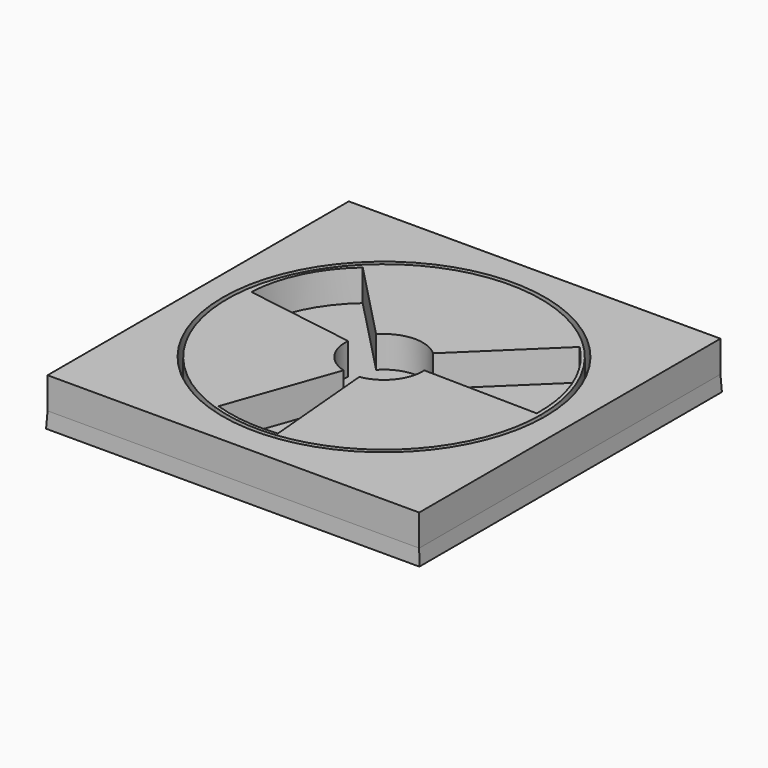
from build123d import *

# Parameters (mm, degrees)
F1_DEPTH  = 12.7
F0_R      = 72.898
F0_R_2    = 65.278
F2_DEPTH  = 12.7
F4_R      = 72.898
F5_DEPTH  = 6.35
F6_DEPTH  = 12.7
F8_W      = 150.4707932472
F8_H      = 152.4543464184
F8_R      = 72.898
F9_DEPTH  = 12.7
F9_FACE_W = 150.4707932472
F9_FACE_H = 152.4543464184
F9_FACE_R = 72.898
F12_DEPTH = 6.35
F12_TAPER = -3


# Not quite as in the source:
# - the program builds the solid bodies; features that only make, move or delete a surface that nothing else refers to are left out


with BuildPart() as f1:
    # F0 (on Top) → F1 (new body)
    with BuildSketch(Plane.XY):
        with BuildLine():
            Line((44.0266140713, 43.9798835084), (44.9402432342, 44.8622841377))
            ThreePointArc((44.9402432342, 44.8622841377), (0.0822011404, 63.499946795), (-44.8239437094, 44.9784845269))
            Line((-44.8239437094, 44.9784845269), (-43.499038361, 43.6043470536))
            Line((-43.499038361, 43.6043470536), (-11.6539793168, 10.5759582539))
            ThreePointArc((-11.6539793168, 10.5759582539), (-0.7689783294, 15.718613146), (10.5660161344, 11.662994039))
            Line((10.5660161344, 11.662994039), (44.0266140713, 43.9798835084))
        make_face()
    extrude(amount=F1_DEPTH)



with BuildPart() as f1b:
    # F0 (on Top) → F1, piece 2 (new body)
    with BuildSketch(Plane.XY):
        with BuildLine():
            ThreePointArc((6.6638546501, -63.1493708694), (47.1891587684, -42.4903906164), (63.4999938049, -0.0280496613))
            Line((63.4999938049, -0.0280496613), (61.8462218281, 0))
            Line((61.8462218281, 0), (15.7179516616, 0.78238256))
            ThreePointArc((15.7179516616, 0.78238256), (12.2084926851, -9.9307015494), (2.4344132667, -15.5479824721))
            Line((2.4344132667, -15.5479824721), (6.5514407483, -61.8841783021))
            Line((6.5514407483, -61.8841783021), (6.6638546501, -63.1493708694))
        make_face()
    extrude(amount=F1_DEPTH)


with BuildPart() as f1c:
    # F0 (on Top) → F1, piece 3 (new body)
    with BuildSketch(Plane.XY):
        with BuildLine():
            Line((-60.5164809282, 8.5368217163), (-62.8717330434, 8.9103975287))
            ThreePointArc((-62.8717330434, 8.9103975287), (-54.0323144536, -33.3580424304), (-20.2050848869, -60.1997055202))
            Line((-20.2050848869, -60.1997055202), (-19.7810930248, -59.0023835005))
            Line((-19.7810930248, -59.0023835005), (-4.2528877081, -15.1518669823))
            ThreePointArc((-4.2528877081, -15.1518669823), (-12.9594991488, -8.928466202), (-15.6728541768, 1.4239974924))
            Line((-15.6728541768, 1.4239974924), (-60.5164809282, 8.5368217163))
        make_face()
    extrude(amount=F1_DEPTH)


with BuildPart() as f2:
    # F0 (on Top) → F2 (new body)
    with BuildSketch(Plane.XY):
        Circle(F0_R)
        Circle(F0_R_2, mode=Mode.SUBTRACT)
    extrude(amount=F2_DEPTH)


with BuildPart() as f1_1:
    add(f1.part)

    add(f1b.part)  # F5 merges F1b

    add(f1c.part)  # F5 merges F1c

    add(f2.part)  # F5 merges F2
    # F4 (on Top) → F5 (join)
    with BuildSketch(Plane.XY):
        Circle(F4_R)
    extrude(amount=-F5_DEPTH)

    # F0 (on Top) → F6 (join)
    with BuildSketch(Plane.XY):
        with BuildLine():
            ThreePointArc((63.4999938049, -0.0280496613), (63.4999984512, -0.014024831), (63.5, 0))
            ThreePointArc((63.5, 0), (58.6768925787, 24.2749310465), (44.9402432342, 44.8622841377))
            Line((44.9402432342, 44.8622841377), (44.0266140713, 43.9798835084))
            ThreePointArc((44.0266140713, 43.9798835084), (50.6520952134, 36.1515995564), (55.9018661031, 27.3414386269))
            ThreePointArc((55.9018661031, 27.3414386269), (60.528045967, 14.0303191282), (61.8462218281, 0))
            Line((61.8462218281, 0), (63.4999938049, -0.0280496613))
        make_face()
        with BuildLine():
            Line((44.0266140713, 43.9798835084), (44.9402432342, 44.8622841377))
            ThreePointArc((44.9402432342, 44.8622841377), (0.0822011404, 63.499946795), (-44.8239437094, 44.9784845269))
            Line((-44.8239437094, 44.9784845269), (-43.499038361, 43.6043470536))
            Line((-43.499038361, 43.6043470536), (-11.6539793168, 10.5759582539))
            ThreePointArc((-11.6539793168, 10.5759582539), (-0.7689783294, 15.718613146), (10.5660161344, 11.662994039))
            Line((10.5660161344, 11.662994039), (44.0266140713, 43.9798835084))
        make_face()
        with BuildLine():
            ThreePointArc((6.6638546501, -63.1493708694), (47.1891587684, -42.4903906164), (63.4999938049, -0.0280496613))
            Line((63.4999938049, -0.0280496613), (61.8462218281, 0))
            Line((61.8462218281, 0), (15.7179516616, 0.78238256))
            ThreePointArc((15.7179516616, 0.78238256), (12.2084926851, -9.9307015494), (2.4344132667, -15.5479824721))
            Line((2.4344132667, -15.5479824721), (6.5514407483, -61.8841783021))
            Line((6.5514407483, -61.8841783021), (6.6638546501, -63.1493708694))
        make_face()
        with BuildLine():
            Line((-43.499038361, 43.6043470536), (-44.8239437094, 44.9784845269))
            ThreePointArc((-44.8239437094, 44.9784845269), (-56.7874671273, 28.4153757192), (-62.8717330434, 8.9103975287))
            Line((-62.8717330434, 8.9103975287), (-60.5164809282, 8.5368217163))
            ThreePointArc((-60.5164809282, 8.5368217163), (-55.6398831968, 27.8331682386), (-43.499038361, 43.6043470536))
        make_face()
        with BuildLine():
            ThreePointArc((-20.2050848869, -60.1997055202), (-6.929383847, -63.1207861128), (6.6638546501, -63.1493708694))
            Line((6.6638546501, -63.1493708694), (6.5514407483, -61.8841783021))
            ThreePointArc((6.5514407483, -61.8841783021), (-6.7699416658, -61.8606562351), (-19.7810930248, -59.0023835005))
            Line((-19.7810930248, -59.0023835005), (-20.2050848869, -60.1997055202))
        make_face()
        with BuildLine():
            Line((-60.5164809282, 8.5368217163), (-62.8717330434, 8.9103975287))
            ThreePointArc((-62.8717330434, 8.9103975287), (-54.0323144536, -33.3580424304), (-20.2050848869, -60.1997055202))
            Line((-20.2050848869, -60.1997055202), (-19.7810930248, -59.0023835005))
            Line((-19.7810930248, -59.0023835005), (-4.2528877081, -15.1518669823))
            ThreePointArc((-4.2528877081, -15.1518669823), (-12.9594991488, -8.928466202), (-15.6728541768, 1.4239974924))
            Line((-15.6728541768, 1.4239974924), (-60.5164809282, 8.5368217163))
        make_face()
    extrude(amount=F6_DEPTH)



with BuildPart() as f6:
    # F0 (on Top) → F6, piece 2 (new body)
    with BuildSketch(Plane.XY):
        Circle(F0_R)
        Circle(F0_R_2, mode=Mode.SUBTRACT)
    extrude(amount=F6_DEPTH)


with BuildPart() as f1_2:
    add(f1_1.part)

    add(f6.part)  # F9 merges F6
    # F8 (on face) → F9 (join)
    with BuildSketch(Plane.XY):
        Rectangle(F8_W, F8_H)
        Circle(F8_R, mode=Mode.SUBTRACT)
    extrude(amount=F9_DEPTH)

    # F9_face (on face) → F12 (join)
    with BuildSketch(Plane(origin=(0, 0, 0), x_dir=(1, 0, 0), z_dir=(0, 0, -1))):
        Rectangle(F9_FACE_W, F9_FACE_H)
        Circle(F9_FACE_R, mode=Mode.SUBTRACT)
    extrude(amount=F12_DEPTH, taper=F12_TAPER)


solid = f1_2.part
